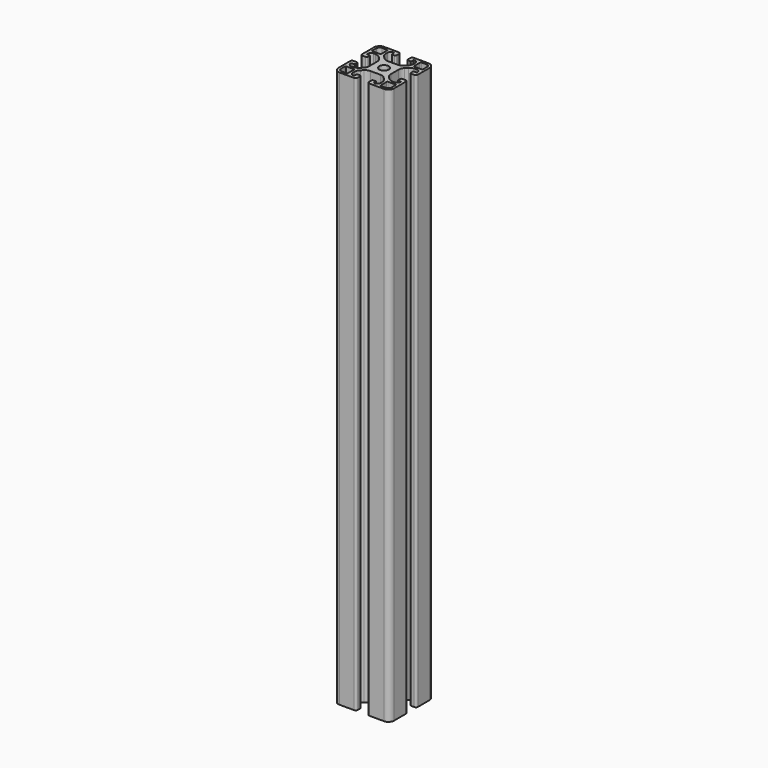
from build123d import *

# Parameters (mm, degrees)
F1_DEPTH = 400


# Not quite as in the source:
# - ends of sketch curves that miss each other by under 0.0002 mm in the source are joined


with BuildPart() as f1:
    # F0 (on Top) → F1 (new body)
    with BuildSketch(Plane.XY):
        with BuildLine():
            Line((7.093145, -9.214466), (8.535534, -10.656855))
            ThreePointArc((8.535534, -10.656855), (9.6193976626, -12.2789708382), (10, -14.192388))
            Line((10, -14.192388), (10, -15.5))
            ThreePointArc((10, -15.5), (9.267766953, -17.267766953), (7.5, -18))
            Line((7.5, -18), (7.450001, -18))
            ThreePointArc((7.450001, -18), (7.1318019485, -17.8681980515), (7, -17.55))
            Line((7, -17.55), (7, -16))
            ThreePointArc((7, -16), (6.8535533906, -15.6464466094), (6.5, -15.5))
            Line((6.5, -15.5), (5, -15.5))
            ThreePointArc((5, -15.5), (4.2928932188, -15.7928932188), (4, -16.5))
            Line((4, -16.5), (4, -18.5))
            ThreePointArc((4, -18.5), (4.4393398282, -19.5606601718), (5.5, -20))
            Line((5.5, -20), (16, -20))
            ThreePointArc((16, -20), (18.8284271247, -18.8284271247), (20, -16))
            Line((20, -16), (20, -5.5))
            ThreePointArc((20, -5.5), (19.5606601718, -4.4393398282), (18.5, -4))
            Line((18.5, -4), (16.5, -4))
            ThreePointArc((16.5, -4), (15.7928932188, -4.2928932188), (15.5, -5))
            Line((15.5, -5), (15.5, -6.5))
            ThreePointArc((15.5, -6.5), (15.6464466094, -6.8535533906), (16, -7))
            Line((16, -7), (17.549999, -7))
            ThreePointArc((17.549999, -7), (17.8681980515, -7.1318019485), (18, -7.45))
            Line((18, -7.45), (18, -7.5))
            ThreePointArc((18, -7.5), (17.267766953, -9.267766953), (15.5, -10))
            Line((15.5, -10), (14.192387, -10))
            ThreePointArc((14.192387, -10), (12.2789708382, -9.6193976626), (10.6568540941, -8.5355339059))
            Line((10.6568540941, -8.5355339059), (9.214466, -7.093145))
            ThreePointArc((9.214466, -7.093145), (8.1306023374, -5.4710291618), (7.75, -3.557612))
            Line((7.75, -3.557612), (7.75, 0))
            Line((7.75, 0), (3.4, 0))
            ThreePointArc((3.4, 0), (2.404163056, -2.404163056), (0, -3.4))
            Line((0, -3.4), (0, -7.75))
            Line((0, -7.75), (3.557611, -7.75))
            ThreePointArc((3.557611, -7.75), (5.4710291618, -8.1306023374), (7.093145, -9.214466))
        make_face()
        with BuildLine():
            Line((16, -18.2), (12.299999, -18.2))
            ThreePointArc((12.299999, -18.2), (11.9464466094, -18.0535533906), (11.8, -17.7))
            Line((11.8, -17.7), (11.799999, -12.3))
            ThreePointArc((11.799999, -12.3), (11.9464466094, -11.9464466094), (12.3, -11.8))
            Line((12.3, -11.8), (17.700001, -11.8))
            ThreePointArc((17.700001, -11.8), (18.0535533906, -11.9464466094), (18.2, -12.3))
            Line((18.2, -12.3), (18.200001, -16))
            ThreePointArc((18.200001, -16), (17.5556349186, -17.5556349186), (16, -18.2))
        make_face(mode=Mode.SUBTRACT)
        with BuildLine():
            Line((-3.557611, -7.75), (0, -7.75))
            Line((0, -7.75), (0, -3.4))
            ThreePointArc((0, -3.4), (-2.404163056, -2.404163056), (-3.4, 0))
            Line((-3.4, 0), (-7.75, 0))
            Line((-7.75, 0), (-7.75, -3.557611))
            ThreePointArc((-7.75, -3.557611), (-8.1306023374, -5.4710291618), (-9.2144660941, -7.0931459059))
            Line((-9.2144660941, -7.0931459059), (-10.656855, -8.535534))
            ThreePointArc((-10.656855, -8.535534), (-12.2789708382, -9.6193976626), (-14.192388, -10))
            Line((-14.192388, -10), (-15.5, -10))
            ThreePointArc((-15.5, -10), (-17.267766953, -9.267766953), (-18, -7.5))
            Line((-18, -7.5), (-18, -7.45))
            ThreePointArc((-18, -7.45), (-17.8681980515, -7.1318019485), (-17.55, -7))
            Line((-17.55, -7), (-16, -7))
            ThreePointArc((-16, -7), (-15.6464466094, -6.8535533906), (-15.5, -6.5))
            Line((-15.5, -6.5), (-15.5, -5))
            ThreePointArc((-15.5, -5), (-15.7928932188, -4.2928932188), (-16.5, -4))
            Line((-16.5, -4), (-18.5, -4))
            ThreePointArc((-18.5, -4), (-19.5606601718, -4.4393398282), (-20, -5.5))
            Line((-20, -5.5), (-20, -16))
            ThreePointArc((-20, -16), (-18.8284271247, -18.8284271247), (-16, -20))
            Line((-16, -20), (-5.5, -20))
            ThreePointArc((-5.5, -20), (-4.4393398282, -19.5606601718), (-4, -18.5))
            Line((-4, -18.5), (-4, -16.5))
            ThreePointArc((-4, -16.5), (-4.2928932188, -15.7928932188), (-5, -15.5))
            Line((-5, -15.5), (-6.5, -15.5))
            ThreePointArc((-6.5, -15.5), (-6.8535533906, -15.6464466094), (-7, -16))
            Line((-7, -16), (-7, -17.55))
            ThreePointArc((-7, -17.55), (-7.1318019485, -17.8681980515), (-7.45, -18))
            Line((-7.45, -18), (-7.5, -18))
            ThreePointArc((-7.5, -18), (-9.267766953, -17.267766953), (-10, -15.5))
            Line((-10, -15.5), (-10, -14.192388))
            ThreePointArc((-10, -14.192388), (-9.6193976626, -12.2789708382), (-8.5355339059, -10.6568540941))
            Line((-8.5355339059, -10.6568540941), (-7.093145, -9.214466))
            ThreePointArc((-7.093145, -9.214466), (-5.4710291618, -8.1306023374), (-3.557611, -7.75))
        make_face()
        with BuildLine():
            Line((-12.3, -18.2), (-16, -18.2))
            ThreePointArc((-16, -18.2), (-17.5556349186, -17.5556349186), (-18.2, -16))
            Line((-18.2, -16), (-18.2, -12.3))
            ThreePointArc((-18.2, -12.3), (-18.0535533906, -11.9464466094), (-17.7, -11.8))
            Line((-17.7, -11.8), (-12.3, -11.8))
            ThreePointArc((-12.3, -11.8), (-11.9464466094, -11.9464466094), (-11.8, -12.3))
            Line((-11.8, -12.3), (-11.8, -17.7))
            ThreePointArc((-11.8, -17.7), (-11.9464466094, -18.0535533906), (-12.3, -18.2))
        make_face(mode=Mode.SUBTRACT)
        with BuildLine():
            Line((-7.75, 0), (-3.4, 0))
            ThreePointArc((-3.4, 0), (-2.404163056, 2.404163056), (0, 3.4))
            Line((0, 3.4), (0, 7.75))
            Line((0, 7.75), (-3.557611, 7.75))
            ThreePointArc((-3.557611, 7.75), (-5.4710291618, 8.1306023374), (-7.0931459059, 9.2144660941))
            Line((-7.0931459059, 9.2144660941), (-8.535534, 10.656855))
            ThreePointArc((-8.535534, 10.656855), (-9.6193976626, 12.2789708382), (-10, 14.192388))
            Line((-10, 14.192388), (-10, 15.5))
            ThreePointArc((-10, 15.5), (-9.267766953, 17.267766953), (-7.5, 18))
            Line((-7.5, 18), (-7.45, 18))
            ThreePointArc((-7.45, 18), (-7.1318019485, 17.8681980515), (-7, 17.55))
            Line((-7, 17.55), (-7, 16))
            ThreePointArc((-7, 16), (-6.8535533906, 15.6464466094), (-6.5, 15.5))
            Line((-6.5, 15.5), (-5, 15.5))
            ThreePointArc((-5, 15.5), (-4.2928932188, 15.7928932188), (-4, 16.5))
            Line((-4, 16.5), (-4, 18.5))
            ThreePointArc((-4, 18.5), (-4.4393398282, 19.5606601718), (-5.5, 20))
            Line((-5.5, 20), (-16, 20))
            ThreePointArc((-16, 20), (-18.8284271247, 18.8284271247), (-20, 16))
            Line((-20, 16), (-20, 5.5))
            ThreePointArc((-20, 5.5), (-19.5606601718, 4.4393398282), (-18.5, 4))
            Line((-18.5, 4), (-16.5, 4))
            ThreePointArc((-16.5, 4), (-15.7928932188, 4.2928932188), (-15.5, 5))
            Line((-15.5, 5), (-15.5, 6.5))
            ThreePointArc((-15.5, 6.5), (-15.6464466094, 6.8535533906), (-16, 7))
            Line((-16, 7), (-17.55, 7))
            ThreePointArc((-17.55, 7), (-17.8681980515, 7.1318019485), (-18, 7.45))
            Line((-18, 7.45), (-18, 7.5))
            ThreePointArc((-18, 7.5), (-17.267766953, 9.267766953), (-15.5, 10))
            Line((-15.5, 10), (-14.192388, 10))
            ThreePointArc((-14.192388, 10), (-12.2789708382, 9.6193976626), (-10.6568540941, 8.5355339059))
            Line((-10.6568540941, 8.5355339059), (-9.214466, 7.093145))
            ThreePointArc((-9.214466, 7.093145), (-8.1306023374, 5.4710291618), (-7.75, 3.557612))
            Line((-7.75, 3.557612), (-7.75, 0))
        make_face()
        with BuildLine():
            Line((-12.3, 11.799999), (-17.7, 11.799999))
            ThreePointArc((-17.7, 11.799999), (-18.0535533906, 11.9464466094), (-18.2, 12.3))
            Line((-18.2, 12.3), (-18.2, 16))
            ThreePointArc((-18.2, 16), (-17.5556349186, 17.5556349186), (-16, 18.2))
            Line((-16, 18.2), (-12.3, 18.200001))
            ThreePointArc((-12.3, 18.200001), (-11.9464466094, 18.0535533906), (-11.8, 17.7))
            Line((-11.8, 17.7), (-11.8, 12.299999))
            ThreePointArc((-11.8, 12.299999), (-11.9464466094, 11.9464466094), (-12.3, 11.799999))
        make_face(mode=Mode.SUBTRACT)
        with BuildLine():
            ThreePointArc((0, 3.4), (2.404163056, 2.404163056), (3.4, 0))
            Line((3.4, 0), (7.75, 0))
            Line((7.75, 0), (7.75, 3.557611))
            ThreePointArc((7.75, 3.557611), (8.1306023374, 5.4710291618), (9.2144660941, 7.0931459059))
            Line((9.2144660941, 7.0931459059), (10.656855, 8.535534))
            ThreePointArc((10.656855, 8.535534), (12.2789708382, 9.6193976626), (14.192388, 10))
            Line((14.192388, 10), (15.5, 10))
            ThreePointArc((15.5, 10), (17.267766953, 9.267766953), (18, 7.5))
            Line((18, 7.5), (18, 7.450001))
            ThreePointArc((18, 7.450001), (17.8681980515, 7.1318019485), (17.55, 7))
            Line((17.55, 7), (16, 7))
            ThreePointArc((16, 7), (15.6464466094, 6.8535533906), (15.5, 6.5))
            Line((15.5, 6.5), (15.5, 5))
            ThreePointArc((15.5, 5), (15.7928932188, 4.2928932188), (16.5, 4))
            Line((16.5, 4), (18.5, 4))
            ThreePointArc((18.5, 4), (19.5606601718, 4.4393398282), (20, 5.5))
            Line((20, 5.5), (20, 16))
            ThreePointArc((20, 16), (18.8284271247, 18.8284271247), (16, 20))
            Line((16, 20), (5.5, 20))
            ThreePointArc((5.5, 20), (4.4393398282, 19.5606601718), (4, 18.5))
            Line((4, 18.5), (4, 16.5))
            ThreePointArc((4, 16.5), (4.2928932188, 15.7928932188), (5, 15.5))
            Line((5, 15.5), (6.5, 15.5))
            ThreePointArc((6.5, 15.5), (6.8535533906, 15.6464466094), (7, 16))
            Line((7, 16), (7, 17.549999))
            ThreePointArc((7, 17.549999), (7.1318019485, 17.8681980515), (7.45, 18))
            Line((7.45, 18), (7.5, 18))
            ThreePointArc((7.5, 18), (9.267766953, 17.267766953), (10, 15.5))
            Line((10, 15.5), (10, 14.192387))
            ThreePointArc((10, 14.192387), (9.6193976626, 12.2789708382), (8.5355339059, 10.6568540941))
            Line((8.5355339059, 10.6568540941), (7.093145, 9.214466))
            ThreePointArc((7.093145, 9.214466), (5.4710291618, 8.1306023374), (3.557612, 7.75))
            Line((3.557612, 7.75), (0, 7.75))
            Line((0, 7.75), (0, 3.4))
        make_face()
        with BuildLine():
            Line((17.700001, 11.799999), (12.299999, 11.799999))
            ThreePointArc((12.299999, 11.799999), (11.9464466094, 11.9464466094), (11.8, 12.3))
            Line((11.8, 12.3), (11.799999, 17.700001))
            ThreePointArc((11.799999, 17.700001), (11.9464466094, 18.0535533906), (12.3, 18.2))
            Line((12.3, 18.2), (16, 18.200001))
            ThreePointArc((16, 18.200001), (17.5556349186, 17.5556349186), (18.2, 16))
            Line((18.2, 16), (18.200001, 12.299999))
            ThreePointArc((18.200001, 12.299999), (18.0535533906, 11.9464466094), (17.700001, 11.799999))
        make_face(mode=Mode.SUBTRACT)
    extrude(amount=F1_DEPTH)


solid = f1.part
